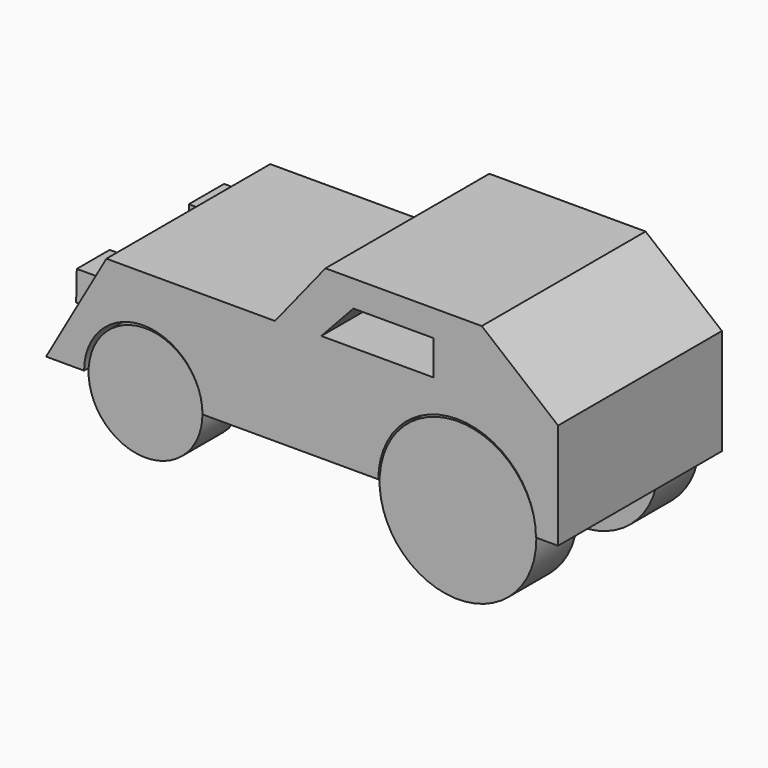
from build123d import *

# Parameters (mm, degrees)
F2_DEPTH  = 50.8
F3_R      = 14.1275934742
F4_DEPTH  = 12.7
F3_R_2    = 19.4394508024
F9_W      = 10.9270086978
F9_H      = 7.2846738622
F10_DEPTH = 58.42


# Not quite as in the source:
# - a feature names something its author has since deleted; it is built from what else it names


with BuildPart() as f2:
    # F1 (on Front) → F2 (new body)
    with BuildSketch(Plane.XZ):
        with BuildLine():
            Line((57.5564166603, 0), (63.0420637049, 0))
            Line((63.0420637049, 0), (63.0420637049, 26.2548112951))
            Line((63.0420637049, 26.2548112951), (44.1141862951, 41.8245235541))
            Line((44.1141862951, 41.8245235541), (5.3425506889, 41.8245235541))
            Line((5.3425506889, 41.8245235541), (-7.1742806475, 26.2548112951))
            Line((-7.1742806475, 26.2548112951), (-48.998799518, 26.2548112951))
            Line((-48.998799518, 26.2548112951), (-63.9579362951, 0))
            Line((-63.9579362951, 0), (-54.5257621315, 0))
            ThreePointArc((-54.5257621315, 0), (-39.8401485541, 14.6856135774), (-25.1545349767, 0))
            Line((-25.1545349767, 0), (18.4604181889, 0))
            ThreePointArc((18.4604181889, 0), (38.0084174246, 19.5479992357), (57.5564166603, 0))
        make_face()
        Polygon((4.302572459, 26.7029106617), (12.2567592189, 35.2952703834), (32.1740247309, 35.2952703834), (32.1740247309, 26.7029106617), align=None, mode=Mode.SUBTRACT)
    extrude(amount=F2_DEPTH)


with BuildPart() as f4:
    # F3 (on Front) → F4 (new body)
    with BuildSketch(Plane.XZ):
        with Locations((-39.7014729679, 0)):
            Circle(F3_R)
    extrude(amount=F4_DEPTH)


with BuildPart() as f4b:
    # F3 (on Front) → F4, piece 2 (new body)
    with BuildSketch(Plane.XZ):
        with Locations((38.0017161369, 0)):
            Circle(F3_R_2)
    extrude(amount=F4_DEPTH)


with BuildPart() as f5_1:
    # F5: copy of F4
    add(f4.part)


with BuildPart() as f7_1:
    # F7: copy of F4b
    add(f4b.part.moved(Location((0, -37.846, -0.508))))


with BuildPart() as f8_1:
    # F8: copy of F4
    add(f4.part.moved(Location((0, -37.592, -0.254))))


with BuildPart() as f10:
    # F9 (on Right) → F10 (new body)
    with BuildSketch(Plane.YZ):
        with Locations((-8.0131421564, 16.2691050209)):
            Rectangle(F9_W, F9_H)
    extrude(amount=-F10_DEPTH)


with BuildPart() as f10b:
    # F9 (on Right) → F10, piece 2 (new body)
    with BuildSketch(Plane.YZ):
        Polygon((-38.0017124116, 19.911441952), (-48.2002533972, 19.911441952), (-48.4008155763, 12.6267680898), (-38.0017124116, 12.6267680898), align=None)
    extrude(amount=-F10_DEPTH)


solid = Compound([f2.part, f4.part, f4b.part, f7_1.part, f8_1.part, f10.part, f10b.part])
